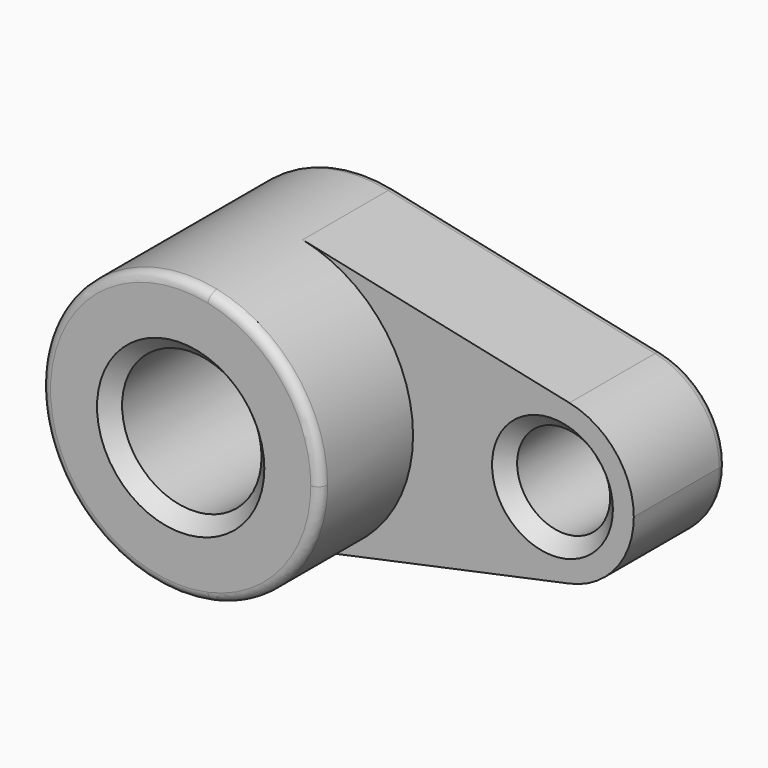
from build123d import *

# Parameters (mm, degrees)
F0_R     = 15
F0_R_2   = 10
F1_DEPTH = 25
F2_DEPTH = 50
F3_R     = 2
F4_SIZE  = 3


# Not quite as in the source:
# - a feature names something its author has since deleted; it is built from what else it names


with BuildPart() as f1:
    # F0 (on Front) → F1 (new body)
    with BuildSketch(Plane.XZ):
        with BuildLine():
            ThreePointArc((6.25, -29.3417364858), (23.3184476327, -18.8745860882), (30, 0))
            ThreePointArc((30, 0), (23.3184476327, 18.8745860882), (6.25, 29.3417364858))
            ThreePointArc((6.25, 29.3417364858), (-30, 0), (6.25, -29.3417364858))
        make_face()
        Circle(F0_R, mode=Mode.SUBTRACT)
        with BuildLine():
            ThreePointArc((6.25, 29.3417364858), (23.3184476327, 18.8745860882), (30, 0))
            ThreePointArc((30, 0), (23.3184476327, -18.8745860882), (6.25, -29.3417364858))
            Line((6.25, -29.3417364858), (63.6458333333, -17.11601295))
            ThreePointArc((63.6458333333, -17.11601295), (42.5, 0), (63.6458333333, 17.11601295))
            Line((63.6458333333, 17.11601295), (6.25, 29.3417364858))
        make_face()
        with BuildLine():
            ThreePointArc((77.5, 0), (73.6024277858, 11.0101752181), (63.6458333333, 17.11601295))
            ThreePointArc((63.6458333333, 17.11601295), (42.5, 0), (63.6458333333, -17.11601295))
            ThreePointArc((63.6458333333, -17.11601295), (73.6024277858, -11.0101752181), (77.5, 0))
        make_face()
        with Locations((60, 0)):
            Circle(F0_R_2, mode=Mode.SUBTRACT)
    extrude(amount=F1_DEPTH)

    # F0 (on Front) → F2 (join)
    with BuildSketch(Plane.XZ):
        with BuildLine():
            ThreePointArc((6.25, -29.3417364858), (23.3184476327, -18.8745860882), (30, 0))
            ThreePointArc((30, 0), (23.3184476327, 18.8745860882), (6.25, 29.3417364858))
            ThreePointArc((6.25, 29.3417364858), (-30, 0), (6.25, -29.3417364858))
        make_face()
        Circle(F0_R, mode=Mode.SUBTRACT)
    extrude(amount=F2_DEPTH)

    # F3
    f3_edges = [f1.edges().sort_by_distance(p)[0] for p in [
        (-6.25, -50, 29.341736),
        (34.947917, 0, -23.228875),
    ]]
    fillet(f3_edges, radius=F3_R)

    # F4
    f4_edges = [f1.edges().sort_by_distance(p)[0] for p in [
        (-15, -50, 0),
        (70, -12.5, 0),
        (50, 0, 0),
        (50, -25, 0),
    ]]
    chamfer(f4_edges, length=F4_SIZE)


solid = f1.part
